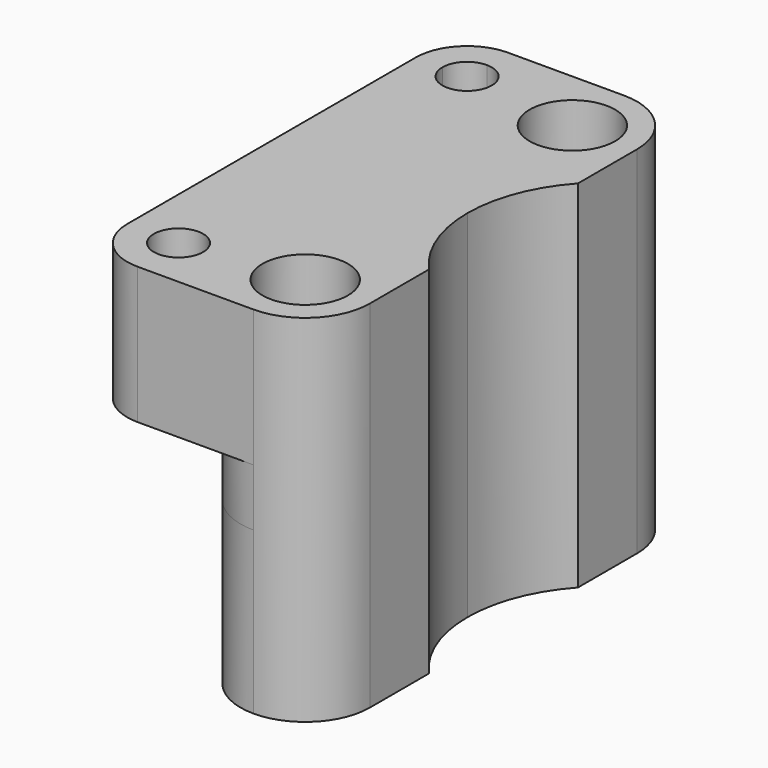
from build123d import *

# Parameters (mm, degrees)
F1_DEPTH = 15
F2_R     = 3.96875
F3_DEPTH = 18.02
F4_R     = 6.002975
F5_R     = 4.7625
F7_DEPTH = 33.02
F8_DEPTH = 5.32


# Not quite as in the source:
# - a fillet or chamfer is up to 0.001 mm smaller than in the source, because OpenCascade refuses the exact size


with BuildPart() as f1:
    # F0 (on Top) → F1 (new body)
    with BuildSketch(Plane.XY):
        Polygon((6.0029852, 0), (0, 0), (0, -43.0059592), (6.0029852, -43.0059592), (12.0059704, -43.0059592), (12.0059704, 0), align=None)
        with BuildLine():
            ThreePointArc((7.5029852, -37.002974), (7.0636453718, -38.0636341718), (6.0029852, -38.502974))
            ThreePointArc((6.0029852, -38.502974), (4.5029852, -37.002974), (6.0029852, -35.502974))
            ThreePointArc((6.0029852, -35.502974), (7.0636453718, -35.9423138282), (7.5029852, -37.002974))
        make_face(mode=Mode.SUBTRACT)
        with BuildLine():
            ThreePointArc((6.0029852, -7.5029852), (4.5029852, -6.0029852), (6.0029852, -4.5029852))
            ThreePointArc((6.0029852, -4.5029852), (7.0636453718, -4.9423250282), (7.5029852, -6.0029852))
            ThreePointArc((7.5029852, -6.0029852), (7.0636453718, -7.0636453718), (6.0029852, -7.5029852))
        make_face(mode=Mode.SUBTRACT)
    extrude(amount=F1_DEPTH)

    # F2 (on face) → F3 (join)
    with BuildSketch(Plane.XY.offset(15)):
        with BuildLine():
            Line((12.0059704, -43.0059592), (12.0059704, 0))
            Line((12.0059704, 0), (-4.7625, 0))
            Line((-4.7625, 0), (-4.7625, -2.4765))
            ThreePointArc((-4.7625, -2.4765), (-3.1460538982, -3.1460538982), (-2.4765, -4.7625))
            ThreePointArc((-2.4765, -4.7625), (-4.7625, -7.0485), (-7.0485, -4.7625))
            Line((-7.0485, -4.7625), (-9.525, -4.7625))
            Line((-9.525, -4.7625), (-9.525, -43.0059592))
            Line((-9.525, -43.0059592), (-4.7625, -43.0059592))
            Line((-4.7625, -43.0059592), (12.0059704, -43.0059592))
        make_face()
        with BuildLine():
            ThreePointArc((-2.4765, -38.2434592), (-3.1460538982, -39.8599053018), (-4.7625, -40.5294592))
            ThreePointArc((-4.7625, -40.5294592), (-6.3789461018, -36.6270130982), (-2.4765, -38.2434592))
        make_face(mode=Mode.SUBTRACT)
        with Locations((6.0029852, -37.002974)):
            Circle(F2_R, mode=Mode.SUBTRACT)
        with Locations((6.0029852, -6.0029852)):
            Circle(F2_R, mode=Mode.SUBTRACT)
        with BuildLine():
            Line((-4.7625, -2.4765), (-4.7625, 0))
            Line((-4.7625, 0), (-9.525, 0))
            Line((-9.525, 0), (-9.525, -4.7625))
            Line((-9.525, -4.7625), (-7.0485, -4.7625))
            ThreePointArc((-7.0485, -4.7625), (-6.3789461018, -3.1460538982), (-4.7625, -2.4765))
        make_face()
    extrude(amount=F3_DEPTH)

    # F4 (radius 6.0029852 in the source; OpenCascade refuses exactly that, so slightly less here)
    f4_edges = [f1.edges().sort_by_distance(p)[0] for p in [
        (12.00597, 0, 16.51),
        (0, 0, 7.5),
        (0, -43.005959, 7.5),
        (12.00597, -43.005959, 16.51),
    ]]
    fillet(f4_edges, radius=F4_R)

    # F5
    f5_edges = [f1.edges().sort_by_distance(p)[0] for p in [
        (-9.525, -43.005959, 24.01),
        (-9.525, 0, 24.01),
    ]]
    fillet(f5_edges, radius=F5_R)

    # F6 (on face) → F7 (cut, through all)
    with BuildSketch(Plane(origin=(0, 0, 0), x_dir=(1, 0, 0), z_dir=(0, 0, -1))):
        with BuildLine():
            ThreePointArc((12.0059704, 30.145029001), (9.5274974569, 26.1361174223), (8.6624922, 21.5029796))
            Line((8.6624922, 21.5029796), (12.0059704, 21.5029796))
            Line((12.0059704, 21.5029796), (12.0059704, 30.145029001))
        make_face()
        with BuildLine():
            Line((12.0059704, 21.5029796), (8.6624922, 21.5029796))
            ThreePointArc((8.6624922, 21.5029796), (9.5274974569, 16.8698417777), (12.0059704, 12.860930199))
            Line((12.0059704, 12.860930199), (12.0059704, 21.5029796))
        make_face()
    extrude(amount=-F7_DEPTH, mode=Mode.SUBTRACT)

    # F8 (cut): a face of the model
    f8_faces = [f1.faces().sort_by_distance(p)[0] for p in [
        (-4.4215962699, -21.5029796, 15),
    ]]
    extrude(f8_faces, amount=-F8_DEPTH, mode=Mode.SUBTRACT)


solid = f1.part
